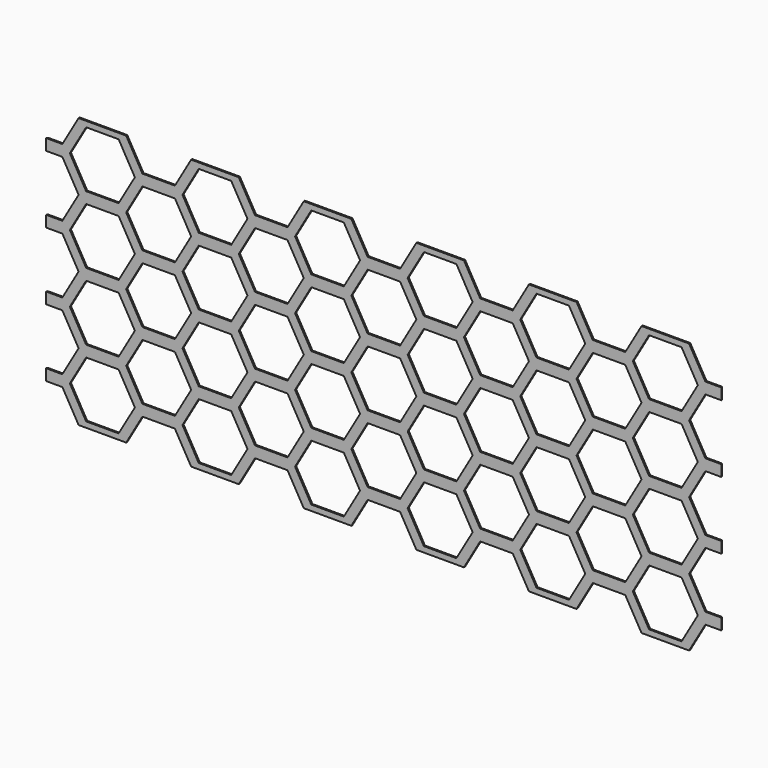
from build123d import *

# Parameters (mm, degrees)
F1_DEPTH    = 3.175
F2_SIZE2    = 1.833077
F2_SIZE     = 3.17499
F3_SIZE2    = 1.833077
F3_SIZE     = 3.17499
F4_SIZE2    = 1.833077
F4_SIZE     = 3.17499
F5_SIZE2    = 1.833077
F5_SIZE     = 3.17499
F6_T1_DEPTH = 41.9033921872
F7_T1_DEPTH = 41.9033921872
F8_T1_DEPTH = 41.9033921872
F9_T1_DEPTH = 41.9033921872


# Not quite as in the source:
# - a fillet or chamfer that OpenCascade refuses, or shapes differently, is made with other operations: its cross-section is extruded or revolved along the edge and cut away or added
# - a fillet or chamfer is up to 0.001 mm smaller than in the source, because OpenCascade refuses the exact size
# - ends of sketch curves that miss each other by under 0.0002 mm in the source are joined


with BuildPart() as f1:
    # F0 (on Front) → F1 (new body)
    with BuildSketch(Plane.XZ):
        Polygon((-350.5809154657, 319.5011963324), (-457.9339551977, 319.5011963324), (-494.5956972913, 256.0012038664), (-531.2574393848, 256.0012038664), (-531.2574393848, 230.6012019829), (-494.5956972913, 230.6012019829), (-457.9339551977, 167.1012019829), (-494.5956972913, 103.6012019829), (-531.2574393848, 103.6012019829), (-531.2574393848, 78.2012000994), (-494.5956972913, 78.2012000994), (-457.9339551977, 14.7012000994), (-494.5956972913, -48.7987999006), (-531.2574393848, -48.7987999006), (-531.2574393848, -74.1988017841), (-494.5956972913, -74.1988017841), (-457.9339551977, -137.6988017841), (-494.5956972913, -201.1988017841), (-531.2574393848, -201.1988017841), (-531.2574393848, -226.5988036676), (-494.5956972913, -226.5988036676), (-457.9339551977, -290.0988036676), (-350.5809154657, -290.0988036676), (-313.9191733721, -226.5988036676), (-240.595689185, -226.5988036676), (-203.9339470915, -290.0988036676), (-96.5809073594, -290.0988036676), (-59.9191652659, -226.5988036676), (13.4043189212, -226.5988036676), (50.0660610147, -290.0988036676), (157.4191007468, -290.0988036676), (194.0808428403, -226.5988036676), (267.4043270274, -226.5988036676), (304.066069121, -290.0988036676), (411.419108853, -290.0988036676), (448.0808509466, -226.5988036676), (521.4043351336, -226.5988036676), (558.0660772272, -290.0988036676), (665.4191169593, -290.0988036676), (702.0808590528, -226.5988036676), (775.4043432399, -226.5988036676), (812.0660853334, -290.0988036676), (919.4191250655, -290.0988036676), (956.080867159, -226.5988036676), (992.7425606152, -226.5988036676), (992.7425606152, -201.1988017841), (956.080867159, -201.1988017841), (919.4191250655, -137.6988017841), (956.080867159, -74.1988017841), (992.7425606152, -74.1988017841), (992.7425606152, -48.7987999006), (956.080867159, -48.7987999006), (919.4191250655, 14.7012000994), (956.080867159, 78.2012000994), (992.7425606152, 78.2012000994), (992.7425606152, 103.6012019829), (956.080867159, 103.6012019829), (919.4191250655, 167.1012019829), (956.080867159, 230.6012019829), (992.7425606152, 230.6012019829), (992.7425606152, 256.0012038664), (956.080867159, 256.0012038664), (919.4191250655, 319.5012038664), (812.0660853334, 319.5011963324), (775.4043432399, 256.0012038664), (702.0808590528, 256.0012038664), (665.4191169593, 319.5012038664), (558.0660772272, 319.5011963324), (521.4043351336, 256.0012038664), (448.0808509466, 256.0012038664), (411.419108853, 319.5012038664), (304.066069121, 319.5011963324), (267.4043270274, 256.0012038664), (194.0808428403, 256.0012038664), (157.4191007468, 319.5012038664), (50.0660610147, 319.5011963324), (13.4043189212, 256.0012038664), (-59.9191652659, 256.0012038664), (-96.5809073594, 319.5012038664), (-203.9339470915, 319.5011963324), (-240.595689185, 256.0012038664), (-313.9191733721, 256.0012038664), align=None)
        Polygon((-477.5809235719, -213.8988036676), (-440.9191814784, -150.3988036676), (-367.5956972913, -150.3988036676), (-330.9339551977, -213.8988036676), (-367.5956972913, -277.3988036676), (-440.9191814784, -277.3988036676), align=None, mode=Mode.SUBTRACT)
        Polygon((-113.595689185, -277.3988036676), (-186.9191733721, -277.3988036676), (-223.5809154657, -213.8988036676), (-186.9191733721, -150.3988036676), (-113.595689185, -150.3988036676), (-76.9339470915, -213.8988036676), align=None, mode=Mode.SUBTRACT)
        Polygon((140.4043189212, -277.3988036676), (67.0808347341, -277.3988036676), (30.4190926406, -213.8988036676), (67.0808347341, -150.3988036676), (140.4043189212, -150.3988036676), (177.0660610147, -213.8988036676), align=None, mode=Mode.SUBTRACT)
        Polygon((-240.595689185, -74.1988017841), (-203.9339470915, -137.6988017841), (-240.595689185, -201.1988017841), (-313.9191733721, -201.1988017841), (-350.5809154657, -137.6988017841), (-313.9191733721, -74.1988017841), align=None, mode=Mode.SUBTRACT)
        Polygon((-367.5956972913, -124.9988017841), (-440.9191814784, -124.9988017841), (-477.5809235719, -61.4988017841), (-440.9191814784, 2.0011982159), (-367.5956972913, 2.0011982159), (-330.9339551977, -61.4988017841), align=None, mode=Mode.SUBTRACT)
        Polygon((13.4043189212, -74.1988017841), (50.0660610147, -137.6988017841), (13.4043189212, -201.1988017841), (-59.9191652659, -201.1988017841), (-96.5809073594, -137.6988017841), (-59.9191652659, -74.1988017841), align=None, mode=Mode.SUBTRACT)
        Polygon((-113.595689185, -124.9988017841), (-186.9191733721, -124.9988017841), (-223.5809154657, -61.4988017841), (-186.9191733721, 2.0011982159), (-113.595689185, 2.0011982159), (-76.9339470915, -61.4988017841), align=None, mode=Mode.SUBTRACT)
        Polygon((13.4043189212, 78.2012000994), (50.0660610147, 14.7012000994), (13.4043189212, -48.7987999006), (-59.9191652659, -48.7987999006), (-96.5809073594, 14.7012000994), (-59.9191652659, 78.2012000994), align=None, mode=Mode.SUBTRACT)
        Polygon((140.4043189212, -124.9988017841), (67.0808347341, -124.9988017841), (30.4190926406, -61.4988017841), (67.0808347341, 2.0011982159), (140.4043189212, 2.0011982159), (177.0660610147, -61.4988017841), align=None, mode=Mode.SUBTRACT)
        Polygon((394.4043270274, -277.3988036676), (321.0808428403, -277.3988036676), (284.4191007468, -213.8988036676), (321.0808428403, -150.3988036676), (394.4043270274, -150.3988036676), (431.066069121, -213.8988036676), align=None, mode=Mode.SUBTRACT)
        Polygon((648.4043351336, -277.3988036676), (575.0808509466, -277.3988036676), (538.419108853, -213.8988036676), (575.0808509466, -150.3988036676), (648.4043351336, -150.3988036676), (685.0660772272, -213.8988036676), align=None, mode=Mode.SUBTRACT)
        Polygon((902.4043432399, -277.3988036676), (829.0808590528, -277.3988036676), (792.4191169593, -213.8988036676), (829.0808590528, -150.3988036676), (902.4043432399, -150.3988036676), (939.0660853334, -213.8988036676), align=None, mode=Mode.SUBTRACT)
        Polygon((267.4043270274, -74.1988017841), (304.066069121, -137.6988017841), (267.4043270274, -201.1988017841), (194.0808428403, -201.1988017841), (157.4191007468, -137.6988017841), (194.0808428403, -74.1988017841), align=None, mode=Mode.SUBTRACT)
        Polygon((521.4043351336, -74.1988017841), (558.0660772272, -137.6988017841), (521.4043351336, -201.1988017841), (448.0808509466, -201.1988017841), (411.419108853, -137.6988017841), (448.0808509466, -74.1988017841), align=None, mode=Mode.SUBTRACT)
        Polygon((394.4043270274, -124.9988017841), (321.0808428403, -124.9988017841), (284.4191007468, -61.4988017841), (321.0808428403, 2.0011982159), (394.4043270274, 2.0011982159), (431.066069121, -61.4988017841), align=None, mode=Mode.SUBTRACT)
        Polygon((267.4043270274, 78.2012000994), (304.066069121, 14.7012000994), (267.4043270274, -48.7987999006), (194.0808428403, -48.7987999006), (157.4191007468, 14.7012000994), (194.0808428403, 78.2012000994), align=None, mode=Mode.SUBTRACT)
        Polygon((648.4043351336, -124.9988017841), (575.0808509466, -124.9988017841), (538.419108853, -61.4988017841), (575.0808509466, 2.0011982159), (648.4043351336, 2.0011982159), (685.0660772272, -61.4988017841), align=None, mode=Mode.SUBTRACT)
        Polygon((521.4043351336, 78.2012000994), (558.0660772272, 14.7012000994), (521.4043351336, -48.7987999006), (448.0808509466, -48.7987999006), (411.419108853, 14.7012000994), (448.0808509466, 78.2012000994), align=None, mode=Mode.SUBTRACT)
        Polygon((775.4043432399, -74.1988017841), (812.0660853334, -137.6988017841), (775.4043432399, -201.1988017841), (702.0808590528, -201.1988017841), (665.4191169593, -137.6988017841), (702.0808590528, -74.1988017841), align=None, mode=Mode.SUBTRACT)
        Polygon((775.4043432399, 78.2012000994), (812.0660853334, 14.7012000994), (775.4043432399, -48.7987999006), (702.0808590528, -48.7987999006), (665.4191169593, 14.7012000994), (702.0808590528, 78.2012000994), align=None, mode=Mode.SUBTRACT)
        Polygon((902.4043432399, -124.9988017841), (829.0808590528, -124.9988017841), (792.4191169593, -61.4988017841), (829.0808590528, 2.0011982159), (902.4043432399, 2.0011982159), (939.0660853334, -61.4988017841), align=None, mode=Mode.SUBTRACT)
        Polygon((-367.5956972913, 27.4012000994), (-440.9191814784, 27.4012000994), (-477.5809235719, 90.9012000994), (-440.9191814784, 154.4012000994), (-367.5956972913, 154.4012000994), (-330.9339551977, 90.9012000994), align=None, mode=Mode.SUBTRACT)
        Polygon((-240.595689185, 78.2012000994), (-203.9339470915, 14.7012000994), (-240.595689185, -48.7987999006), (-313.9191733721, -48.7987999006), (-350.5809154657, 14.7012000994), (-313.9191733721, 78.2012000994), align=None, mode=Mode.SUBTRACT)
        Polygon((-240.595689185, 230.6012019829), (-203.9339470915, 167.1012019829), (-240.595689185, 103.6012019829), (-313.9191733721, 103.6012019829), (-350.5809154657, 167.1012019829), (-313.9191733721, 230.6012019829), align=None, mode=Mode.SUBTRACT)
        Polygon((-113.595689185, 27.4012000994), (-186.9191733721, 27.4012000994), (-223.5809154657, 90.9012000994), (-186.9191733721, 154.4012000994), (-113.595689185, 154.4012000994), (-76.9339470915, 90.9012000994), align=None, mode=Mode.SUBTRACT)
        Polygon((140.4043189212, 27.4012000994), (67.0808347341, 27.4012000994), (30.4190926406, 90.9012000994), (67.0808347341, 154.4012000994), (140.4043189212, 154.4012000994), (177.0660610147, 90.9012000994), align=None, mode=Mode.SUBTRACT)
        Polygon((13.4043189212, 230.6012019829), (50.0660610147, 167.1012019829), (13.4043189212, 103.6012019829), (-59.9191652659, 103.6012019829), (-96.5809073594, 167.1012019829), (-59.9191652659, 230.6012019829), align=None, mode=Mode.SUBTRACT)
        Polygon((-367.5956972913, 179.8012019829), (-440.9191814784, 179.8012019829), (-477.5809235719, 243.3012019829), (-440.9191814784, 306.8012019829), (-367.5956972913, 306.8012019829), (-330.9339551977, 243.3012019829), align=None, mode=Mode.SUBTRACT)
        Polygon((-113.595689185, 179.8012019829), (-186.9191733721, 179.8012019829), (-223.5809154657, 243.3012019829), (-186.9191733721, 306.8012019829), (-113.595689185, 306.8012019829), (-76.9339470915, 243.3012019829), align=None, mode=Mode.SUBTRACT)
        Polygon((140.4043189212, 179.8012019829), (67.0808347341, 179.8012019829), (30.4190926406, 243.3012019829), (67.0808347341, 306.8012019829), (140.4043189212, 306.8012019829), (177.0660610147, 243.3012019829), align=None, mode=Mode.SUBTRACT)
        Polygon((394.4043270274, 27.4012000994), (321.0808428403, 27.4012000994), (284.4191007468, 90.9012000994), (321.0808428403, 154.4012000994), (394.4043270274, 154.4012000994), (431.066069121, 90.9012000994), align=None, mode=Mode.SUBTRACT)
        Polygon((648.4043351336, 27.4012000994), (575.0808509466, 27.4012000994), (538.419108853, 90.9012000994), (575.0808509466, 154.4012000994), (648.4043351336, 154.4012000994), (685.0660772272, 90.9012000994), align=None, mode=Mode.SUBTRACT)
        Polygon((267.4043270274, 230.6012019829), (304.066069121, 167.1012019829), (267.4043270274, 103.6012019829), (194.0808428403, 103.6012019829), (157.4191007468, 167.1012019829), (194.0808428403, 230.6012019829), align=None, mode=Mode.SUBTRACT)
        Polygon((521.4043351336, 230.6012019829), (558.0660772272, 167.1012019829), (521.4043351336, 103.6012019829), (448.0808509466, 103.6012019829), (411.419108853, 167.1012019829), (448.0808509466, 230.6012019829), align=None, mode=Mode.SUBTRACT)
        Polygon((902.4043432399, 27.4012000994), (829.0808590528, 27.4012000994), (792.4191169593, 90.9012000994), (829.0808590528, 154.4012000994), (902.4043432399, 154.4012000994), (939.0660853334, 90.9012000994), align=None, mode=Mode.SUBTRACT)
        Polygon((775.4043432399, 230.6012019829), (812.0660853334, 167.1012019829), (775.4043432399, 103.6012019829), (702.0808590528, 103.6012019829), (665.4191169593, 167.1012019829), (702.0808590528, 230.6012019829), align=None, mode=Mode.SUBTRACT)
        Polygon((394.4043270274, 179.8012019829), (321.0808428403, 179.8012019829), (284.4191007468, 243.3012019829), (321.0808428403, 306.8012019829), (394.4043270274, 306.8012019829), (431.066069121, 243.3012019829), align=None, mode=Mode.SUBTRACT)
        Polygon((648.4043351336, 179.8012019829), (575.0808509466, 179.8012019829), (538.419108853, 243.3012019829), (575.0808509466, 306.8012019829), (648.4043351336, 306.8012019829), (685.0660772272, 243.3012019829), align=None, mode=Mode.SUBTRACT)
        Polygon((902.4043432399, 179.8012019829), (829.0808590528, 179.8012019829), (792.4191169593, 243.3012019829), (829.0808590528, 306.8012019829), (902.4043432399, 306.8012019829), (939.0660853334, 243.3012019829), align=None, mode=Mode.SUBTRACT)
    extrude(amount=F1_DEPTH)

    # F2 (size 3.175 and 1.8330871047 in the source; OpenCascade refuses exactly that, so slightly less here)
    f2_edges = [f1.edges().sort_by_distance(p)[0] for p in [
        (-531.257439, 0, 243.301203),
    ]]
    f2_side = f1.faces().sort_by_distance((-531.257439, -1.5875, 243.301203))[0]
    chamfer(f2_edges, length=F2_SIZE, length2=F2_SIZE2, reference=f2_side)

    # F3 (size 3.175 and 1.8330871047 in the source; OpenCascade refuses exactly that, so slightly less here)
    f3_edges = [f1.edges().sort_by_distance(p)[0] for p in [
        (-531.257439, 0, 90.901201),
    ]]
    f3_side = f1.faces().sort_by_distance((-531.257439, -1.5875, 90.901201))[0]
    chamfer(f3_edges, length=F3_SIZE, length2=F3_SIZE2, reference=f3_side)

    # F4 (size 3.175 and 1.8330871047 in the source; OpenCascade refuses exactly that, so slightly less here)
    f4_edges = [f1.edges().sort_by_distance(p)[0] for p in [
        (-531.257439, 0, -61.498801),
    ]]
    f4_side = f1.faces().sort_by_distance((-531.257439, -1.5875, -61.498801))[0]
    chamfer(f4_edges, length=F4_SIZE, length2=F4_SIZE2, reference=f4_side)

    # F5 (size 3.175 and 1.8330871047 in the source; OpenCascade refuses exactly that, so slightly less here)
    f5_edges = [f1.edges().sort_by_distance(p)[0] for p in [
        (-531.257439, 0, -213.898803),
    ]]
    f5_side = f1.faces().sort_by_distance((-531.257439, -1.5875, -213.898803))[0]
    chamfer(f5_edges, length=F5_SIZE, length2=F5_SIZE2, reference=f5_side)

    # F6: chamfer of 1.8415 x 3.1895715621 on 1 edges, made by hand

    # F6_s2 → F6_t1 (cut)
    with BuildSketch(Plane.XY.offset(222.3495068311)):
        Polygon((990.9010606152, 0), (992.7425606152, -3.1895715621), (992.7425606152, 0), align=None)
    extrude(amount=F6_T1_DEPTH, mode=Mode.SUBTRACT)

    # F7: chamfer of 1.8415 x 3.1895715621 on 1 edges, made by hand

    # F7_s2 → F7_t1 (cut)
    with BuildSketch(Plane.XY.offset(69.9495049476)):
        Polygon((990.9010606152, 0), (992.7425606152, -3.1895715621), (992.7425606152, 0), align=None)
    extrude(amount=F7_T1_DEPTH, mode=Mode.SUBTRACT)

    # F8: chamfer of 1.8415 x 3.1895715621 on 1 edges, made by hand

    # F8_s2 → F8_t1 (cut)
    with BuildSketch(Plane.XY.offset(-82.4504969359)):
        Polygon((990.9010606152, 0), (992.7425606152, -3.1895715621), (992.7425606152, 0), align=None)
    extrude(amount=F8_T1_DEPTH, mode=Mode.SUBTRACT)

    # F9: chamfer of 1.8415 x 3.1895715621 on 1 edges, made by hand

    # F9_s2 → F9_t1 (cut)
    with BuildSketch(Plane.XY.offset(-234.8504988194)):
        Polygon((990.9010606152, 0), (992.7425606152, -3.1895715621), (992.7425606152, 0), align=None)
    extrude(amount=F9_T1_DEPTH, mode=Mode.SUBTRACT)


solid = f1.part
